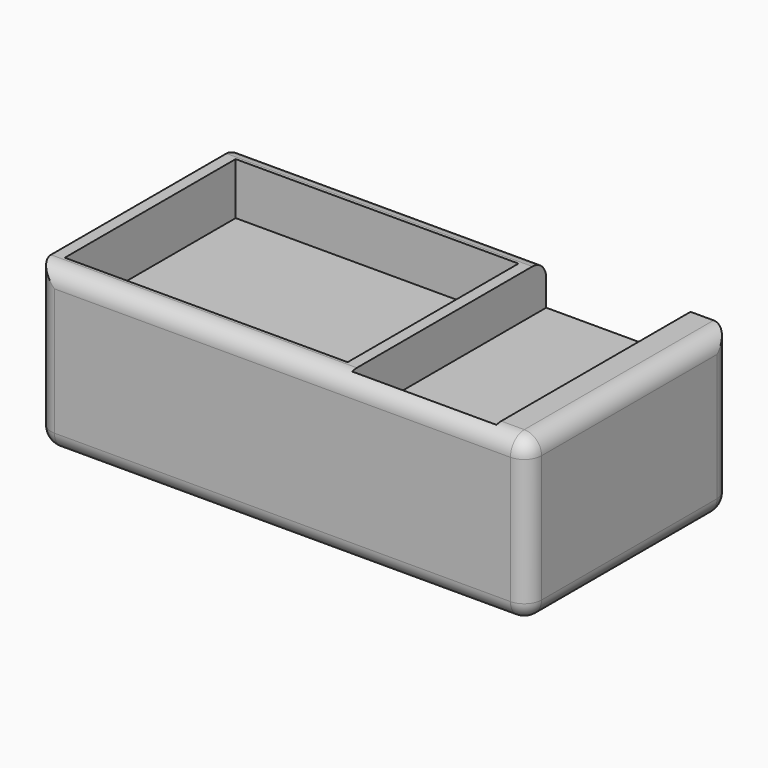
from build123d import *

# Parameters (mm, degrees)
F0_W         = 85
F0_H         = 44
F1_DEPTH     = 28
F2_W         = 49
F2_H         = 37
F3_DEPTH     = 9
F2_W_2       = 25
F2_H_2       = 42
F4_DEPTH     = 7.5
F5_W         = 25
F5_H         = 13
F5_R         = 1.25
F6_DEPTH     = 16
F7_T1_DEPTH  = 22
F7_T3_DEPTH  = 32.5
F7_T5_DEPTH  = 79
F7_T7_DEPTH  = 38
F7_T9_DEPTH  = 68
F7_T11_DEPTH = 89.5
F7_T13_DEPTH = 48.5
F7_S17_W     = 3
F7_S17_H     = 3
F7_T18_DEPTH = 3
F7_S23_W     = 3
F7_S23_H     = 3
F7_T24_DEPTH = 3
F7_S29_W     = 3
F7_S29_H     = 3
F7_T30_DEPTH = 3
F7_S35_W     = 3
F7_S35_H     = 3
F7_T36_DEPTH = 3
F7_S41_W     = 3
F7_S41_H     = 3
F7_T42_DEPTH = 3


# Not quite as in the source:
# - a fillet or chamfer that OpenCascade refuses, or shapes differently, is made with other operations: its cross-section is extruded or revolved along the edge and cut away or added


with BuildPart() as f1:
    # F0 (on Top) → F1 (new body)
    with BuildSketch(Plane.XY):
        with Locations((12.7505162358, -9.2363715138)):
            Rectangle(F0_W, F0_H)
    extrude(amount=F1_DEPTH)

    # F2 (on face) → F3 (cut)
    with BuildSketch(Plane.XY.offset(28)):
        with Locations((-3.2494837642, -9.2363715138)):
            Rectangle(F2_W, F2_H)
    extrude(amount=-F3_DEPTH, mode=Mode.SUBTRACT)

    # F2 (on face) → F4 (cut)
    with BuildSketch(Plane.XY.offset(28)):
        with Locations((35.7505162358, -8.2363715138)):
            Rectangle(F2_W_2, F2_H_2)
    extrude(amount=-F4_DEPTH, mode=Mode.SUBTRACT)

    # F5 (on face) → F6 (cut)
    with BuildSketch(Plane(origin=(0, 0, 0), x_dir=(1, 0, 0), z_dir=(0, 0, -1))):
        with Locations((-12.2494837642, 9.2363715138)):
            Rectangle(F5_W, F5_H)
        with Locations((37.7505162358, 9.2363715138)):
            Rectangle(F5_W, F5_H)
        with Locations((-26.9994837642, 9.2363715138)):
            Circle(F5_R)
        with Locations((2.5005162358, 9.2363715138)):
            Circle(F5_R)
        with Locations((23.0005162358, 9.2363715138)):
            Circle(F5_R)
        with Locations((52.5005162358, 9.2363715138)):
            Circle(F5_R)
    extrude(amount=-F6_DEPTH, mode=Mode.SUBTRACT)

    # F7: fillet of radius 3 on 11 edges, made by hand

    # F7_s2 → F7_t1 (cut)
    with BuildSketch(Plane.XY.offset(3)):
        with BuildLine():
            ThreePointArc((55.2505162358, -28.2363715138), (54.3718365794, -30.3576918574), (52.2505162358, -31.2363715138))
            Line((52.2505162358, -31.2363715138), (55.2505162358, -31.2363715138))
            Line((55.2505162358, -31.2363715138), (55.2505162358, -28.2363715138))
        make_face()
    extrude(amount=F7_T1_DEPTH, mode=Mode.SUBTRACT)

    # F7_s4 → F7_t3 (cut)
    with BuildSketch(Plane.XY.offset(3)):
        with BuildLine():
            ThreePointArc((52.2505162358, 12.7636284862), (54.3718365794, 11.8849488297), (55.2505162358, 9.7636284862))
            Line((55.2505162358, 9.7636284862), (55.2505162358, 12.7636284862))
            Line((55.2505162358, 12.7636284862), (52.2505162358, 12.7636284862))
        make_face()
        with BuildLine():
            ThreePointArc((-29.7494837642, -28.2363715138), (-28.8708041077, -30.3576918574), (-26.7494837642, -31.2363715138))
            Line((-26.7494837642, -31.2363715138), (-29.7494837642, -31.2363715138))
            Line((-29.7494837642, -31.2363715138), (-29.7494837642, -28.2363715138))
        make_face()
        with BuildLine():
            ThreePointArc((-26.7494837642, 12.7636284862), (-28.8708041077, 11.8849488297), (-29.7494837642, 9.7636284862))
            Line((-29.7494837642, 9.7636284862), (-29.7494837642, 12.7636284862))
            Line((-29.7494837642, 12.7636284862), (-26.7494837642, 12.7636284862))
        make_face()
    extrude(amount=F7_T3_DEPTH, mode=Mode.SUBTRACT)

    # F7_s6 → F7_t5 (cut)
    with BuildSketch(Plane.YZ.offset(-26.7494837642)):
        with BuildLine():
            ThreePointArc((12.7636284862, 3), (11.8849488297, 0.8786796564), (9.7636284862, 0))
            Line((9.7636284862, 0), (12.7636284862, 0))
            Line((12.7636284862, 0), (12.7636284862, 3))
        make_face()
        with BuildLine():
            ThreePointArc((-28.2363715138, 0), (-30.3576918574, 0.8786796564), (-31.2363715138, 3))
            Line((-31.2363715138, 3), (-31.2363715138, 0))
            Line((-31.2363715138, 0), (-28.2363715138, 0))
        make_face()
    extrude(amount=F7_T5_DEPTH, mode=Mode.SUBTRACT)

    # F7_s8 → F7_t7 (cut)
    with BuildSketch(Plane.XZ.offset(-9.7636284862)):
        with BuildLine():
            ThreePointArc((-26.7494837642, 0), (-28.8708041077, 0.8786796564), (-29.7494837642, 3))
            Line((-29.7494837642, 3), (-29.7494837642, 0))
            Line((-29.7494837642, 0), (-26.7494837642, 0))
        make_face()
        with BuildLine():
            ThreePointArc((52.2505162358, 0), (54.3718365794, 0.8786796564), (55.2505162358, 3))
            Line((55.2505162358, 3), (55.2505162358, 0))
            Line((55.2505162358, 0), (52.2505162358, 0))
        make_face()
    extrude(amount=F7_T7_DEPTH, mode=Mode.SUBTRACT)

    # F7_s10 → F7_t9 (cut)
    with BuildSketch(Plane.YZ.offset(-37.2494837642)):
        with BuildLine():
            ThreePointArc((12.7636284862, 25), (11.8849488297, 27.1213203436), (9.7636284862, 28))
            Line((9.7636284862, 28), (12.7636284862, 28))
            Line((12.7636284862, 28), (12.7636284862, 25))
        make_face()
    extrude(amount=F7_T9_DEPTH, mode=Mode.SUBTRACT)

    # F7_s12 → F7_t11 (cut)
    with BuildSketch(Plane.YZ.offset(-37.2494837642)):
        with BuildLine():
            ThreePointArc((-28.2363715138, 28), (-30.3576918574, 27.1213203436), (-31.2363715138, 25))
            Line((-31.2363715138, 25), (-31.2363715138, 28))
            Line((-31.2363715138, 28), (-28.2363715138, 28))
        make_face()
    extrude(amount=F7_T11_DEPTH, mode=Mode.SUBTRACT)

    # F7_s14 → F7_t13 (cut)
    with BuildSketch(Plane.XZ.offset(-20.2636284862)):
        with BuildLine():
            ThreePointArc((52.2505162358, 28), (54.3718365794, 27.1213203436), (55.2505162358, 25))
            Line((55.2505162358, 25), (55.2505162358, 28))
            Line((55.2505162358, 28), (52.2505162358, 28))
        make_face()
    extrude(amount=F7_T13_DEPTH, mode=Mode.SUBTRACT)


with BuildPart() as f7_tool16:
    # F7_s17 → F7_t18 (new body)
    with BuildSketch(Plane.XZ.offset(28.2363715138)):
        with Locations((53.7505162358, 1.5)):
            Rectangle(F7_S17_W, F7_S17_H)
    extrude(amount=F7_T18_DEPTH)

    # F7_s19 → F7_t20 (revolve, cut)
    with BuildSketch(Plane(origin=(52.2505162358, -28.2363715138, 3), x_dir=(-0.7071067812, 0, 0.7071067812), z_dir=(0.7071067812, 0, 0.7071067812))):
        with BuildLine():
            ThreePointArc((0, -3), (3, 0), (0, 3))
            Line((0, 3), (0, -3))
        make_face()
    revolve(axis=Axis((52.2505162358, -28.2363715138, 3), (0, -1, 0)), mode=Mode.SUBTRACT)


with BuildPart() as f1_1:
    add(f1.part)

    # F7_t15: cut F7_tool16
    add(f7_tool16.part, mode=Mode.SUBTRACT)


with BuildPart() as f7_tool22:
    # F7_s23 → F7_t24 (new body)
    with BuildSketch(Plane.XZ.offset(28.2363715138)):
        with Locations((53.7505162358, 26.5)):
            Rectangle(F7_S23_W, F7_S23_H)
    extrude(amount=F7_T24_DEPTH)

    # F7_s25 → F7_t26 (revolve, cut)
    with BuildSketch(Plane(origin=(52.2505162358, -28.2363715138, 25), x_dir=(-0.7071067812, 0, -0.7071067812), z_dir=(-0.7071067812, 0, 0.7071067812))):
        with BuildLine():
            ThreePointArc((0, -3), (3, 0), (0, 3))
            Line((0, 3), (0, -3))
        make_face()
    revolve(axis=Axis((52.2505162358, -28.2363715138, 25), (0, -1, 0)), mode=Mode.SUBTRACT)


with BuildPart() as f1_2:
    add(f1_1.part)

    # F7_t21: cut F7_tool22
    add(f7_tool22.part, mode=Mode.SUBTRACT)


with BuildPart() as f7_tool28:
    # F7_s29 → F7_t30 (new body)
    with BuildSketch(Plane.XZ.offset(-9.7636284862)):
        with Locations((53.7505162358, 1.5)):
            Rectangle(F7_S29_W, F7_S29_H)
    extrude(amount=-F7_T30_DEPTH)

    # F7_s31 → F7_t32 (revolve, cut)
    with BuildSketch(Plane(origin=(52.2505162358, 9.7636284862, 3), x_dir=(-0.7071067812, 0, 0.7071067812), z_dir=(-0.7071067812, 0, -0.7071067812))):
        with BuildLine():
            ThreePointArc((0, -3), (3, 0), (0, 3))
            Line((0, 3), (0, -3))
        make_face()
    revolve(axis=Axis((52.2505162358, 9.7636284862, 3), (0, 1, 0)), mode=Mode.SUBTRACT)


with BuildPart() as f1_3:
    add(f1_2.part)

    # F7_t27: cut F7_tool28
    add(f7_tool28.part, mode=Mode.SUBTRACT)


with BuildPart() as f7_tool34:
    # F7_s35 → F7_t36 (new body)
    with BuildSketch(Plane.XZ.offset(28.2363715138)):
        with Locations((-28.2494837642, 1.5)):
            Rectangle(F7_S35_W, F7_S35_H)
    extrude(amount=F7_T36_DEPTH)

    # F7_s37 → F7_t38 (revolve, cut)
    with BuildSketch(Plane(origin=(-26.7494837642, -28.2363715138, 3), x_dir=(0.7071067812, 0, 0.7071067812), z_dir=(0.7071067812, 0, -0.7071067812))):
        with BuildLine():
            ThreePointArc((0, -3), (3, 0), (0, 3))
            Line((0, 3), (0, -3))
        make_face()
    revolve(axis=Axis((-26.7494837642, -28.2363715138, 3), (0, -1, 0)), mode=Mode.SUBTRACT)


with BuildPart() as f1_4:
    add(f1_3.part)

    # F7_t33: cut F7_tool34
    add(f7_tool34.part, mode=Mode.SUBTRACT)


with BuildPart() as f7_tool40:
    # F7_s41 → F7_t42 (new body)
    with BuildSketch(Plane.XZ.offset(-9.7636284862)):
        with Locations((-28.2494837642, 1.5)):
            Rectangle(F7_S41_W, F7_S41_H)
    extrude(amount=-F7_T42_DEPTH)

    # F7_s43 → F7_t44 (revolve, cut)
    with BuildSketch(Plane(origin=(-26.7494837642, 9.7636284862, 3), x_dir=(0.7071067812, 0, 0.7071067812), z_dir=(-0.7071067812, 0, 0.7071067812))):
        with BuildLine():
            ThreePointArc((0, -3), (3, 0), (0, 3))
            Line((0, 3), (0, -3))
        make_face()
    revolve(axis=Axis((-26.7494837642, 9.7636284862, 3), (0, 1, 0)), mode=Mode.SUBTRACT)


with BuildPart() as f1_5:
    add(f1_4.part)

    # F7_t39: cut F7_tool40
    add(f7_tool40.part, mode=Mode.SUBTRACT)


solid = f1_5.part
